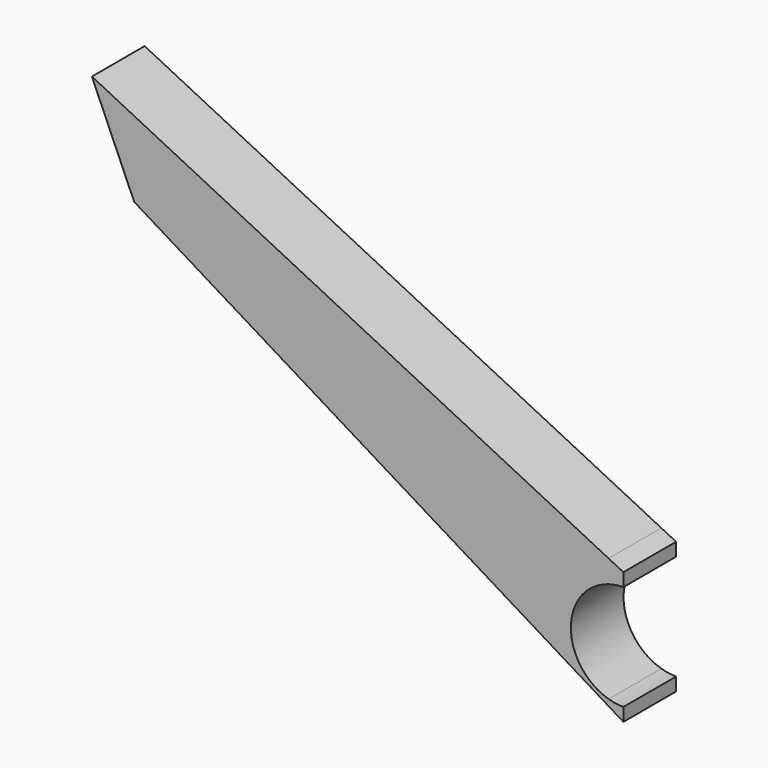
from build123d import *

# Parameters (mm, degrees)
F1_DEPTH = 6.35


# Not quite as in the source:
# - a feature names something its author has since deleted; it is built from what else it names


with BuildPart() as f1:
    # F0 (on Front) → F1 (new body)
    with BuildSketch(Plane.XZ):
        with BuildLine():
            Line((-5.7584308088, -7.4710633766), (-4.3362458402, -8.3395278))
            Line((-4.3362458402, -8.3395278), (-4.3362458402, -7.0695278))
            ThreePointArc((-4.3362458402, -7.0695278), (-5.054777107, -7.0154621069), (-5.7584308088, -6.8602791556))
            Line((-5.7584308088, -6.8602791556), (-5.7584308088, -7.4710633766))
        make_face()
        with BuildLine():
            ThreePointArc((-5.7584308088, 2.8812235555), (-5.054777107, 3.0364065068), (-4.3362458402, 3.0904722))
            Line((-4.3362458402, 3.0904722), (-4.3362458402, 4.3604722))
            Line((-4.3362458402, 4.3604722), (-5.7584308088, 5.0656502469))
            Line((-5.7584308088, 5.0656502469), (-5.7584308088, 2.8812235555))
        make_face()
        with BuildLine():
            Line((-51.4653283692, 20.4400841292), (-5.7584308088, -7.4710633766))
            Line((-5.7584308088, -7.4710633766), (-5.7584308088, -6.8602791556))
            ThreePointArc((-5.7584308088, -6.8602791556), (-9.3953454824, -1.9895278), (-5.7584308088, 2.8812235555))
            Line((-5.7584308088, 2.8812235555), (-5.7584308088, 5.0656502469))
            Line((-5.7584308088, 5.0656502469), (-55.5376484304, 29.7482423422))
            Line((-55.5376484304, 29.7482423422), (-51.4653283692, 20.4400841292))
        make_face()
    extrude(amount=F1_DEPTH)


solid = f1.part
